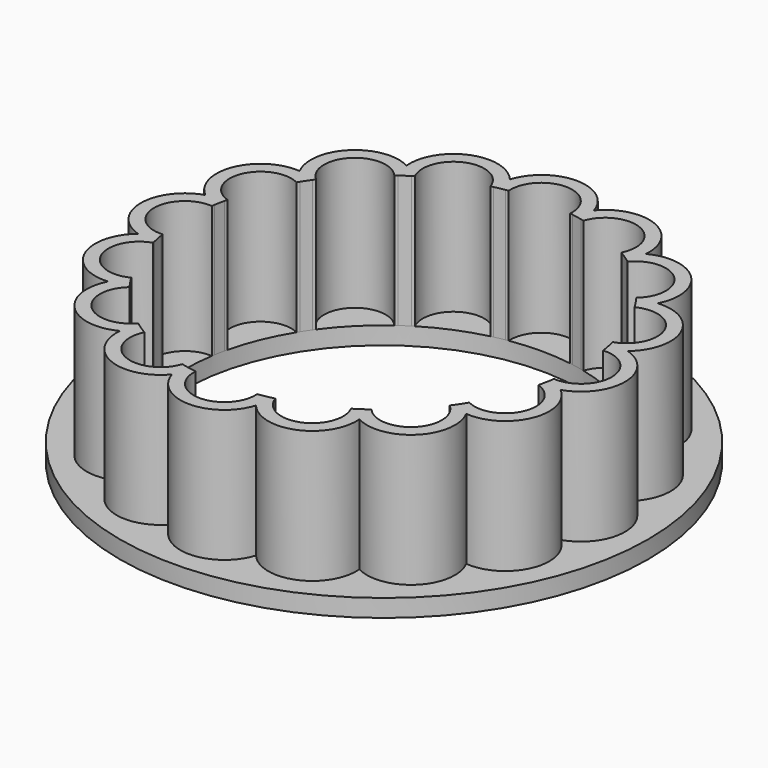
from build123d import *

# Parameters (mm, degrees)
F0_R     = 30
F0_R_2   = 22.5
F1_DEPTH = 2
F3_DEPTH = 15


# Not quite as in the source:
# - after a boolean that leaves OpenCascade's solid faulty, fix() repairs it


with BuildPart() as f1:
    # F0 (on Top) → F1 (new body)
    with BuildSketch(Plane.XY):
        with Locations((0, 0.1543397957)):
            Circle(F0_R)
        Circle(F0_R_2, mode=Mode.SUBTRACT)
    extrude(amount=F1_DEPTH)

    # F2 (on face) → F3 (join)
    with BuildSketch(Plane.XY.offset(2)):
        with BuildLine():
            ThreePointArc((-3.8069810153, 22.1755923382), (-3.6482825778, 22.2022529089), (-3.4893975213, 22.2277777778))
            ThreePointArc((-3.4893975213, 22.2277777778), (0, 26), (3.4893975213, 22.2277777778))
            ThreePointArc((3.4893975213, 22.2277777778), (3.6482825778, 22.2022529089), (3.8069810153, 22.1755923382))
            ThreePointArc((3.8069810153, 22.1755923382), (4.1952253001, 23.1338685771), (4.7722662453, 23.991802562))
            ThreePointArc((4.7722662453, 23.991802562), (0, 27.5), (-4.7722662453, 23.991802562))
            ThreePointArc((-4.7722662453, 23.991802562), (-4.1952253001, 23.1338685771), (-3.8069810153, 22.1755923382))
        make_face()
        with BuildLine():
            ThreePointArc((-4.96903995, 21.9444444444), (-4.3895322454, 22.0676688091), (-3.8069810153, 22.1755923382))
            ThreePointArc((-3.8069810153, 22.1755923382), (-4.1952253001, 23.1338685771), (-4.7722662453, 23.991802562))
            ThreePointArc((-4.7722662453, 23.991802562), (-4.9770654419, 22.9783509036), (-4.96903995, 21.9444444444))
        make_face()
        with BuildLine():
            ThreePointArc((-5.2824193431, 21.8711235624), (-5.125860747, 21.9083443373), (-4.96903995, 21.9444444444))
            ThreePointArc((-4.96903995, 21.9444444444), (-4.9770654419, 22.9783509036), (-4.7722662453, 23.991802562))
            ThreePointArc((-4.7722662453, 23.991802562), (-10.52379439, 25.4066871441), (-13.5902644608, 20.3392681081))
            ThreePointArc((-13.5902644608, 20.3392681081), (-12.72883102, 19.7674644688), (-12.0034236314, 19.0307073207))
            ThreePointArc((-12.0034236314, 19.0307073207), (-11.8670079519, 19.1160697391), (-11.7299852446, 19.2004543218))
            ThreePointArc((-11.7299852446, 19.2004543218), (-9.9497692415, 24.0208678453), (-5.2824193431, 21.8711235624))
        make_face()
        with BuildLine():
            ThreePointArc((4.7722662453, 23.991802562), (4.1952253001, 23.1338685771), (3.8069810153, 22.1755923382))
            ThreePointArc((3.8069810153, 22.1755923382), (4.3895322454, 22.0676688091), (4.96903995, 21.9444444444))
            ThreePointArc((4.96903995, 21.9444444444), (4.9770654419, 22.9783509036), (4.7722662453, 23.991802562))
        make_face()
        with BuildLine():
            ThreePointArc((13.5902644608, 20.3392681081), (10.52379439, 25.4066871441), (4.7722662453, 23.991802562))
            ThreePointArc((4.7722662453, 23.991802562), (4.9770654419, 22.9783509036), (4.96903995, 21.9444444444))
            ThreePointArc((4.96903995, 21.9444444444), (5.125860747, 21.9083443373), (5.2824193431, 21.8711235624))
            ThreePointArc((5.2824193431, 21.8711235624), (9.9497692415, 24.0208678453), (11.7299852446, 19.2004543218))
            ThreePointArc((11.7299852446, 19.2004543218), (11.8670079519, 19.1160697391), (12.0034236314, 19.0307073207))
            ThreePointArc((12.0034236314, 19.0307073207), (12.72883102, 19.7674644688), (13.5902644608, 20.3392681081))
        make_face()
        with BuildLine():
            ThreePointArc((-12.0034236314, 19.0307073207), (-12.72883102, 19.7674644688), (-13.5902644608, 20.3392681081))
            ThreePointArc((-13.5902644608, 20.3392681081), (-13.3916430876, 19.3245876043), (-12.9885696274, 18.3724538109))
            ThreePointArc((-12.9885696274, 18.3724538109), (-12.5003302429, 18.7080662768), (-12.0034236314, 19.0307073207))
        make_face()
        with BuildLine():
            ThreePointArc((-12.9885696274, 18.3724538109), (-13.3916430876, 19.3245876043), (-13.5902644608, 20.3392681081))
            ThreePointArc((-13.5902644608, 20.3392681081), (-19.4454364826, 19.4454364826), (-20.3392681081, 13.5902644608))
            ThreePointArc((-20.3392681081, 13.5902644608), (-19.3245876043, 13.3916430876), (-18.3724538109, 12.9885696274))
            ThreePointArc((-18.3724538109, 12.9885696274), (-18.27908894, 13.1196382391), (-18.1847890469, 13.2500357478))
            ThreePointArc((-18.1847890469, 13.2500357478), (-18.3847763109, 18.3847763109), (-13.2500357478, 18.1847890469))
            ThreePointArc((-13.2500357478, 18.1847890469), (-13.1196382391, 18.27908894), (-12.9885696274, 18.3724538109))
        make_face()
        with BuildLine():
            ThreePointArc((12.9885696274, 18.3724538109), (13.3916430876, 19.3245876043), (13.5902644608, 20.3392681081))
            ThreePointArc((13.5902644608, 20.3392681081), (12.72883102, 19.7674644688), (12.0034236314, 19.0307073207))
            ThreePointArc((12.0034236314, 19.0307073207), (12.5003302429, 18.7080662768), (12.9885696274, 18.3724538109))
        make_face()
        with BuildLine():
            ThreePointArc((20.3392681081, 13.5902644608), (19.4454364826, 19.4454364826), (13.5902644608, 20.3392681081))
            ThreePointArc((13.5902644608, 20.3392681081), (13.3916430876, 19.3245876043), (12.9885696274, 18.3724538109))
            ThreePointArc((12.9885696274, 18.3724538109), (13.1196382391, 18.27908894), (13.2500357478, 18.1847890469))
            ThreePointArc((13.2500357478, 18.1847890469), (18.3847763109, 18.3847763109), (18.1847890469, 13.2500357478))
            ThreePointArc((18.1847890469, 13.2500357478), (18.27908894, 13.1196382391), (18.3724538109, 12.9885696274))
            ThreePointArc((18.3724538109, 12.9885696274), (19.3245876043, 13.3916430876), (20.3392681081, 13.5902644608))
        make_face()
        with BuildLine():
            ThreePointArc((-18.3724538109, 12.9885696274), (-19.3245876043, 13.3916430876), (-20.3392681081, 13.5902644608))
            ThreePointArc((-20.3392681081, 13.5902644608), (-19.7674644688, 12.72883102), (-19.0307073207, 12.0034236314))
            ThreePointArc((-19.0307073207, 12.0034236314), (-18.7080662768, 12.5003302429), (-18.3724538109, 12.9885696274))
        make_face()
        with BuildLine():
            ThreePointArc((-19.0307073207, 12.0034236314), (-19.7674644688, 12.72883102), (-20.3392681081, 13.5902644608))
            ThreePointArc((-20.3392681081, 13.5902644608), (-25.4066871441, 10.52379439), (-23.991802562, 4.7722662453))
            ThreePointArc((-23.991802562, 4.7722662453), (-22.9783509036, 4.9770654419), (-21.9444444444, 4.96903995))
            ThreePointArc((-21.9444444444, 4.96903995), (-21.9083443373, 5.125860747), (-21.8711235624, 5.2824193431))
            ThreePointArc((-21.8711235624, 5.2824193431), (-24.0208678453, 9.9497692415), (-19.2004543218, 11.7299852446))
            ThreePointArc((-19.2004543218, 11.7299852446), (-19.1160697391, 11.8670079519), (-19.0307073207, 12.0034236314))
        make_face()
        with BuildLine():
            ThreePointArc((19.0307073207, 12.0034236314), (19.7674644688, 12.72883102), (20.3392681081, 13.5902644608))
            ThreePointArc((20.3392681081, 13.5902644608), (19.3245876043, 13.3916430876), (18.3724538109, 12.9885696274))
            ThreePointArc((18.3724538109, 12.9885696274), (18.7080662768, 12.5003302429), (19.0307073207, 12.0034236314))
        make_face()
        with BuildLine():
            ThreePointArc((23.991802562, 4.7722662453), (25.4066871441, 10.52379439), (20.3392681081, 13.5902644608))
            ThreePointArc((20.3392681081, 13.5902644608), (19.7674644688, 12.72883102), (19.0307073207, 12.0034236314))
            ThreePointArc((19.0307073207, 12.0034236314), (19.1160697391, 11.8670079519), (19.2004543218, 11.7299852446))
            ThreePointArc((19.2004543218, 11.7299852446), (24.0208678453, 9.9497692415), (21.8711235624, 5.2824193431))
            ThreePointArc((21.8711235624, 5.2824193431), (21.9083443373, 5.125860747), (21.9444444444, 4.96903995))
            ThreePointArc((21.9444444444, 4.96903995), (22.9783509036, 4.9770654419), (23.991802562, 4.7722662453))
        make_face()
        with BuildLine():
            ThreePointArc((-21.9444444444, 4.96903995), (-22.9783509036, 4.9770654419), (-23.991802562, 4.7722662453))
            ThreePointArc((-23.991802562, 4.7722662453), (-23.1338685771, 4.1952253001), (-22.1755923382, 3.8069810153))
            ThreePointArc((-22.1755923382, 3.8069810153), (-22.0676688091, 4.3895322454), (-21.9444444444, 4.96903995))
        make_face()
        with BuildLine():
            ThreePointArc((-22.1755923382, 3.8069810153), (-23.1338685771, 4.1952253001), (-23.991802562, 4.7722662453))
            ThreePointArc((-23.991802562, 4.7722662453), (-27.5, 0), (-23.991802562, -4.7722662453))
            ThreePointArc((-23.991802562, -4.7722662453), (-23.1338685771, -4.1952253001), (-22.1755923382, -3.8069810153))
            ThreePointArc((-22.1755923382, -3.8069810153), (-22.2022529089, -3.6482825778), (-22.2277777778, -3.4893975213))
            ThreePointArc((-22.2277777778, -3.4893975213), (-26, 0), (-22.2277777778, 3.4893975213))
            ThreePointArc((-22.2277777778, 3.4893975213), (-22.2022529089, 3.6482825778), (-22.1755923382, 3.8069810153))
        make_face()
        with BuildLine():
            ThreePointArc((22.1755923382, 3.8069810153), (23.1338685771, 4.1952253001), (23.991802562, 4.7722662453))
            ThreePointArc((23.991802562, 4.7722662453), (22.9783509036, 4.9770654419), (21.9444444444, 4.96903995))
            ThreePointArc((21.9444444444, 4.96903995), (22.0676688091, 4.3895322454), (22.1755923382, 3.8069810153))
        make_face()
        with BuildLine():
            ThreePointArc((23.991802562, -4.7722662453), (27.5, 0), (23.991802562, 4.7722662453))
            ThreePointArc((23.991802562, 4.7722662453), (23.1338685771, 4.1952253001), (22.1755923382, 3.8069810153))
            ThreePointArc((22.1755923382, 3.8069810153), (22.2022529089, 3.6482825778), (22.2277777778, 3.4893975213))
            ThreePointArc((22.2277777778, 3.4893975213), (26, 0), (22.2277777778, -3.4893975213))
            ThreePointArc((22.2277777778, -3.4893975213), (22.2022529089, -3.6482825778), (22.1755923382, -3.8069810153))
            ThreePointArc((22.1755923382, -3.8069810153), (23.1338685771, -4.1952253001), (23.991802562, -4.7722662453))
        make_face()
        with BuildLine():
            ThreePointArc((-22.1755923382, -3.8069810153), (-23.1338685771, -4.1952253001), (-23.991802562, -4.7722662453))
            ThreePointArc((-23.991802562, -4.7722662453), (-22.9783509036, -4.9770654419), (-21.9444444444, -4.96903995))
            ThreePointArc((-21.9444444444, -4.96903995), (-22.0676688091, -4.3895322454), (-22.1755923382, -3.8069810153))
        make_face()
        with BuildLine():
            ThreePointArc((-21.9444444444, -4.96903995), (-22.9783509036, -4.9770654419), (-23.991802562, -4.7722662453))
            ThreePointArc((-23.991802562, -4.7722662453), (-25.4066871441, -10.52379439), (-20.3392681081, -13.5902644608))
            ThreePointArc((-20.3392681081, -13.5902644608), (-19.7674644688, -12.72883102), (-19.0307073207, -12.0034236314))
            ThreePointArc((-19.0307073207, -12.0034236314), (-19.1160697391, -11.8670079519), (-19.2004543218, -11.7299852446))
            ThreePointArc((-19.2004543218, -11.7299852446), (-24.0208678453, -9.9497692415), (-21.8711235624, -5.2824193431))
            ThreePointArc((-21.8711235624, -5.2824193431), (-21.9083443373, -5.125860747), (-21.9444444444, -4.96903995))
        make_face()
        with BuildLine():
            ThreePointArc((21.9444444444, -4.96903995), (22.9783509036, -4.9770654419), (23.991802562, -4.7722662453))
            ThreePointArc((23.991802562, -4.7722662453), (23.1338685771, -4.1952253001), (22.1755923382, -3.8069810153))
            ThreePointArc((22.1755923382, -3.8069810153), (22.0676688091, -4.3895322454), (21.9444444444, -4.96903995))
        make_face()
        with BuildLine():
            ThreePointArc((20.3392681081, -13.5902644608), (25.4066871441, -10.52379439), (23.991802562, -4.7722662453))
            ThreePointArc((23.991802562, -4.7722662453), (22.9783509036, -4.9770654419), (21.9444444444, -4.96903995))
            ThreePointArc((21.9444444444, -4.96903995), (21.9083443373, -5.125860747), (21.8711235624, -5.2824193431))
            ThreePointArc((21.8711235624, -5.2824193431), (24.0208678453, -9.9497692415), (19.2004543218, -11.7299852446))
            ThreePointArc((19.2004543218, -11.7299852446), (19.1160697391, -11.8670079519), (19.0307073207, -12.0034236314))
            ThreePointArc((19.0307073207, -12.0034236314), (19.7674644688, -12.72883102), (20.3392681081, -13.5902644608))
        make_face()
        with BuildLine():
            ThreePointArc((-19.0307073207, -12.0034236314), (-19.7674644688, -12.72883102), (-20.3392681081, -13.5902644608))
            ThreePointArc((-20.3392681081, -13.5902644608), (-19.3245876043, -13.3916430876), (-18.3724538109, -12.9885696274))
            ThreePointArc((-18.3724538109, -12.9885696274), (-18.7080662768, -12.5003302429), (-19.0307073207, -12.0034236314))
        make_face()
        with BuildLine():
            ThreePointArc((-18.3724538109, -12.9885696274), (-19.3245876043, -13.3916430876), (-20.3392681081, -13.5902644608))
            ThreePointArc((-20.3392681081, -13.5902644608), (-19.4454364826, -19.4454364826), (-13.5902644608, -20.3392681081))
            ThreePointArc((-13.5902644608, -20.3392681081), (-13.3916430876, -19.3245876043), (-12.9885696274, -18.3724538109))
            ThreePointArc((-12.9885696274, -18.3724538109), (-13.1196382391, -18.27908894), (-13.2500357478, -18.1847890469))
            ThreePointArc((-13.2500357478, -18.1847890469), (-18.3847763109, -18.3847763109), (-18.1847890469, -13.2500357478))
            ThreePointArc((-18.1847890469, -13.2500357478), (-18.27908894, -13.1196382391), (-18.3724538109, -12.9885696274))
        make_face()
        with BuildLine():
            ThreePointArc((18.3724538109, -12.9885696274), (19.3245876043, -13.3916430876), (20.3392681081, -13.5902644608))
            ThreePointArc((20.3392681081, -13.5902644608), (19.7674644688, -12.72883102), (19.0307073207, -12.0034236314))
            ThreePointArc((19.0307073207, -12.0034236314), (18.7080662768, -12.5003302429), (18.3724538109, -12.9885696274))
        make_face()
        with BuildLine():
            ThreePointArc((13.5902644608, -20.3392681081), (19.4454364826, -19.4454364826), (20.3392681081, -13.5902644608))
            ThreePointArc((20.3392681081, -13.5902644608), (19.3245876043, -13.3916430876), (18.3724538109, -12.9885696274))
            ThreePointArc((18.3724538109, -12.9885696274), (18.27908894, -13.1196382391), (18.1847890469, -13.2500357478))
            ThreePointArc((18.1847890469, -13.2500357478), (18.3847763109, -18.3847763109), (13.2500357478, -18.1847890469))
            ThreePointArc((13.2500357478, -18.1847890469), (13.1196382391, -18.27908894), (12.9885696274, -18.3724538109))
            ThreePointArc((12.9885696274, -18.3724538109), (13.3916430876, -19.3245876043), (13.5902644608, -20.3392681081))
        make_face()
        with BuildLine():
            ThreePointArc((-12.9885696274, -18.3724538109), (-13.3916430876, -19.3245876043), (-13.5902644608, -20.3392681081))
            ThreePointArc((-13.5902644608, -20.3392681081), (-12.72883102, -19.7674644688), (-12.0034236314, -19.0307073207))
            ThreePointArc((-12.0034236314, -19.0307073207), (-12.5003302429, -18.7080662768), (-12.9885696274, -18.3724538109))
        make_face()
        with BuildLine():
            ThreePointArc((-12.0034236314, -19.0307073207), (-12.72883102, -19.7674644688), (-13.5902644608, -20.3392681081))
            ThreePointArc((-13.5902644608, -20.3392681081), (-10.52379439, -25.4066871441), (-4.7722662453, -23.991802562))
            ThreePointArc((-4.7722662453, -23.991802562), (-4.9770654419, -22.9783509036), (-4.96903995, -21.9444444444))
            ThreePointArc((-4.96903995, -21.9444444444), (-5.125860747, -21.9083443373), (-5.2824193431, -21.8711235624))
            ThreePointArc((-5.2824193431, -21.8711235624), (-9.9497692415, -24.0208678453), (-11.7299852446, -19.2004543218))
            ThreePointArc((-11.7299852446, -19.2004543218), (-11.8670079519, -19.1160697391), (-12.0034236314, -19.0307073207))
        make_face()
        with BuildLine():
            ThreePointArc((12.0034236314, -19.0307073207), (12.72883102, -19.7674644688), (13.5902644608, -20.3392681081))
            ThreePointArc((13.5902644608, -20.3392681081), (13.3916430876, -19.3245876043), (12.9885696274, -18.3724538109))
            ThreePointArc((12.9885696274, -18.3724538109), (12.5003302429, -18.7080662768), (12.0034236314, -19.0307073207))
        make_face()
        with BuildLine():
            ThreePointArc((4.7722662453, -23.991802562), (10.52379439, -25.4066871441), (13.5902644608, -20.3392681081))
            ThreePointArc((13.5902644608, -20.3392681081), (12.72883102, -19.7674644688), (12.0034236314, -19.0307073207))
            ThreePointArc((12.0034236314, -19.0307073207), (11.8670079519, -19.1160697391), (11.7299852446, -19.2004543218))
            ThreePointArc((11.7299852446, -19.2004543218), (9.9497692415, -24.0208678453), (5.2824193431, -21.8711235624))
            ThreePointArc((5.2824193431, -21.8711235624), (5.125860747, -21.9083443373), (4.96903995, -21.9444444444))
            ThreePointArc((4.96903995, -21.9444444444), (4.9770654419, -22.9783509036), (4.7722662453, -23.991802562))
        make_face()
        with BuildLine():
            ThreePointArc((-4.96903995, -21.9444444444), (-4.9770654419, -22.9783509036), (-4.7722662453, -23.991802562))
            ThreePointArc((-4.7722662453, -23.991802562), (-4.1952253001, -23.1338685771), (-3.8069810153, -22.1755923382))
            ThreePointArc((-3.8069810153, -22.1755923382), (-4.3895322454, -22.0676688091), (-4.96903995, -21.9444444444))
        make_face()
        with BuildLine():
            ThreePointArc((-3.8069810153, -22.1755923382), (-4.1952253001, -23.1338685771), (-4.7722662453, -23.991802562))
            ThreePointArc((-4.7722662453, -23.991802562), (0, -27.5), (4.7722662453, -23.991802562))
            ThreePointArc((4.7722662453, -23.991802562), (4.1952253001, -23.1338685771), (3.8069810153, -22.1755923382))
            ThreePointArc((3.8069810153, -22.1755923382), (3.6482825778, -22.2022529089), (3.4893975213, -22.2277777778))
            ThreePointArc((3.4893975213, -22.2277777778), (0, -26), (-3.4893975213, -22.2277777778))
            ThreePointArc((-3.4893975213, -22.2277777778), (-3.6482825778, -22.2022529089), (-3.8069810153, -22.1755923382))
        make_face()
        with BuildLine():
            ThreePointArc((3.8069810153, -22.1755923382), (4.1952253001, -23.1338685771), (4.7722662453, -23.991802562))
            ThreePointArc((4.7722662453, -23.991802562), (4.9770654419, -22.9783509036), (4.96903995, -21.9444444444))
            ThreePointArc((4.96903995, -21.9444444444), (4.3895322454, -22.0676688091), (3.8069810153, -22.1755923382))
        make_face()
    extrude(amount=F3_DEPTH)

    add(f1.part.fix(), mode=Mode.REPLACE)


solid = f1.part
